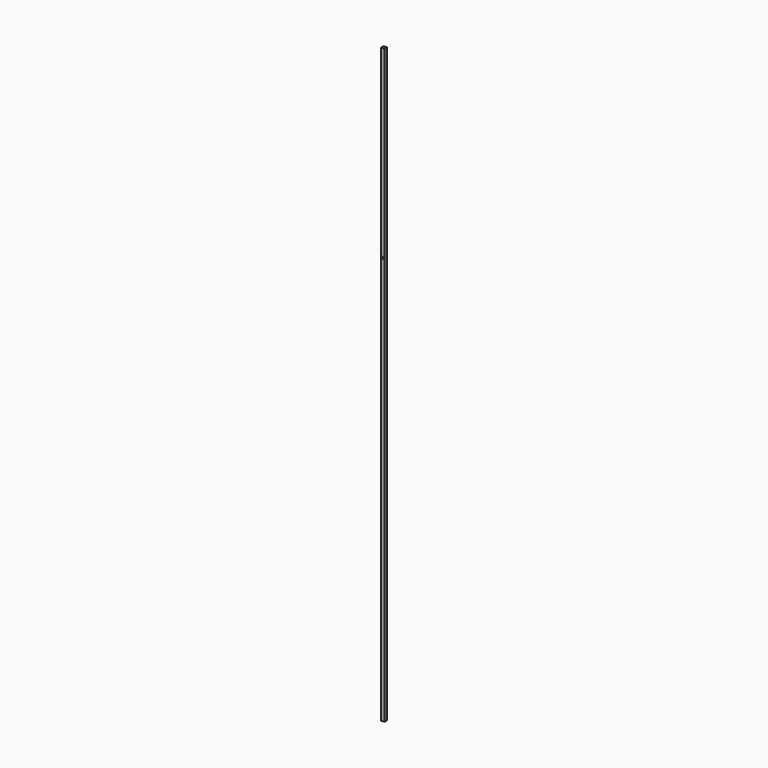
from build123d import *

# Parameters (mm, degrees)
F0_W     = 5
F0_H     = 950
F0_R     = 1.5
F1_DEPTH = 5


# Not quite as in the source:
# - a feature names something its author has since deleted; it is built from what else it names


with BuildPart() as f1:
    # F0 (on Front) → F1 (new body)
    with BuildSketch(Plane.XZ):
        with Locations((-59.2914944887, 508.6652547121)):
            Rectangle(F0_W, F0_H)
        with Locations((-59.5406442881, 687.6652547121)):
            Circle(F0_R, mode=Mode.SUBTRACT)
    extrude(amount=F1_DEPTH)


solid = f1.part
